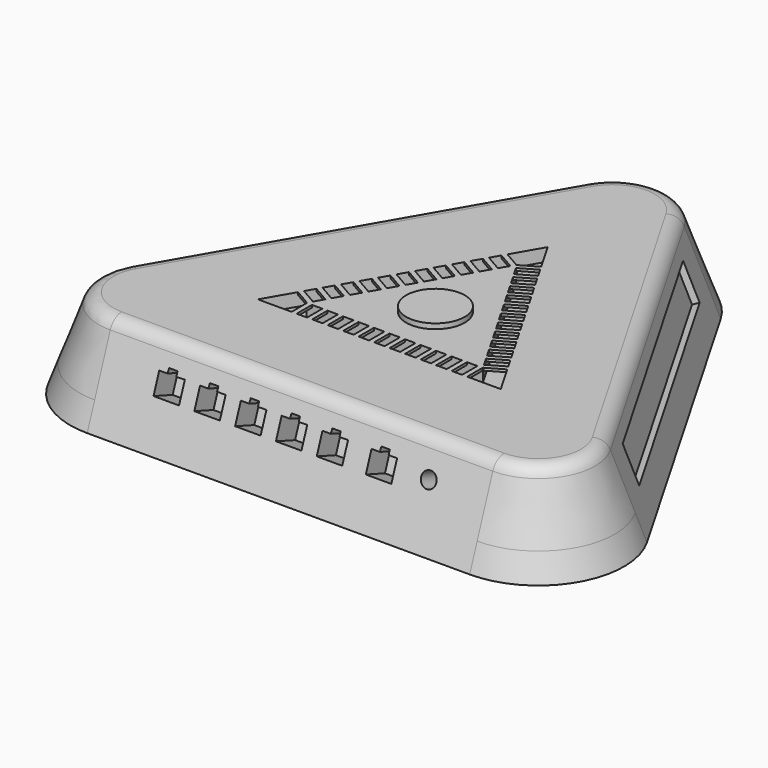
from build123d import *

# Parameters (mm, degrees)
F1_DEPTH      = 25
F1_TAPER      = 20
F1_DEPTH_BACK = 10
F1_TAPER_BACK = -20
F2_R          = 6
F3_R          = 11.5
F4_DEPTH      = 2
F6_R          = 13.9278343954
F7_DEPTH      = 3
F8_R          = 32.5
F9_DEPTH      = 5
F10_R         = 3
F11_DEPTH     = 2
F13_DEPTH     = 5
F15_W         = 1.9796080887
F15_H         = 8.6034480482
F16_DEPTH     = 1
F17_DEPTH     = 10
F19_DEPTH     = 2.5


with BuildPart() as f1:
    # F0 (on Top) → F1 (new body, two sides)
    with BuildSketch(Plane.XY) as f1_sk:
        with BuildLine():
            Line((-75, -73.3012701892), (75, -73.3012701892))
            ThreePointArc((75, -73.3012701892), (100.9807621135, -58.3012701892), (100.9807621135, -28.3012701892))
            Line((100.9807621135, -28.3012701892), (25.9807621135, 101.6025403784))
            ThreePointArc((25.9807621135, 101.6025403784), (0, 116.6025403784), (-25.9807621135, 101.6025403784))
            Line((-25.9807621135, 101.6025403784), (-100.9807621135, -28.3012701892))
            ThreePointArc((-100.9807621135, -28.3012701892), (-100.9807621135, -58.3012701892), (-75, -73.3012701892))
        make_face()
    extrude(amount=F1_DEPTH, taper=F1_TAPER)
    extrude(f1_sk.sketch, amount=-F1_DEPTH_BACK, taper=F1_TAPER_BACK)

    # F2
    f2_edges = [f1.edges().sort_by_distance(p)[0] for p in [
        (-93.100575, -53.751642, 25),
        (0, -64.202014, 25),
        (93.100575, -53.751642, 25),
        (55.600575, 32.101007, 25),
        (0, 107.503285, 25),
        (-55.600575, 32.101007, 25),
    ]]
    fillet(f2_edges, radius=F2_R)

    # F3 (on face) → F4 (join)
    with BuildSketch(Plane.XY.offset(25)):
        Circle(F3_R)
    extrude(amount=F4_DEPTH)

    # F6 (on face) → F7 (join)
    with BuildSketch(Plane(origin=(0, 0, -10), x_dir=(1, 0, 0), z_dir=(0, 0, -1))):
        with Locations((-79.5582754758, 42.91382827)):
            Circle(F6_R)
        with Locations((79.5582754758, 42.91382827)):
            Circle(F6_R)
        with Locations((0, -90.3564020991)):
            Circle(F6_R)
    extrude(amount=F7_DEPTH)

    # F8 (on face) → F9 (cut)
    with BuildSketch(Plane(origin=(0, 0, -10), x_dir=(1, 0, 0), z_dir=(0, 0, -1))):
        Circle(F8_R)
    extrude(amount=-F9_DEPTH, mode=Mode.SUBTRACT)

    # F10 (on face) → F11 (cut)
    with BuildSketch(Plane(origin=(0, -64.7266504456, 23.558574126), x_dir=(1, 0, 0), z_dir=(0, -0.9396926208, 0.3420201433))):
        Polygon((-53.9876961336, -9.3026818497), (-53.9876961336, -17.5021458417), (-43.9876961336, -17.5021458417), (-43.9579116181, -9.2383237345), (-47.2984413058, -9.3026818497), (-47.2984413058, -7.5021458417), (-50.609186478, -7.5021458417), (-50.7396796718, -9.3026818497), align=None)
        Polygon((-34.7396796718, -9.3026818497), (-37.9876961336, -9.3026818497), (-37.9876961336, -17.5021458417), (-27.9876961336, -17.5021458417), (-27.9579116181, -9.2383237345), (-31.2984413058, -9.3026818497), (-31.2984413058, -7.5021458417), (-34.609186478, -7.5021458417), align=None)
        Polygon((-18.7396796718, -9.3026818497), (-21.9876961336, -9.3026818497), (-21.9876961336, -17.5021458417), (-11.9876961336, -17.5021458417), (-11.9579116181, -9.2383237345), (-15.2984413058, -9.3026818497), (-15.2984413058, -7.5021458417), (-18.609186478, -7.5021458417), align=None)
        Polygon((-2.7396796718, -9.3026818497), (-5.9876961336, -9.3026818497), (-5.9876961336, -17.5021458417), (4.0123038664, -17.5021458417), (4.0420883819, -9.2383237345), (0.7015586942, -9.3026818497), (0.7015586942, -7.5021458417), (-2.609186478, -7.5021458417), align=None)
        Polygon((13.2603203282, -9.3026818497), (10.0123038664, -9.3026818497), (10.0123038664, -17.5021458417), (20.0123038664, -17.5021458417), (20.0420883819, -9.2383237345), (16.7015586942, -9.3026818497), (16.7015586942, -7.5021458417), (13.390813522, -7.5021458417), align=None)
        Polygon((32.5083367899, -9.3026819218), (29.2603203282, -9.3026819218), (29.2603203282, -17.5021459138), (39.2603203282, -17.5021459138), (39.2901048437, -9.2383238067), (35.949575156, -9.3026819218), (35.949575156, -7.5021459138), (32.6388299838, -7.5021459138), align=None)
        with Locations((52.4860955775, -12.1968975291)):
            Circle(F10_R)
    extrude(amount=-F11_DEPTH, mode=Mode.SUBTRACT)

    # F3 (on face) → F13 (cut)
    with BuildSketch(Plane.XY.offset(25)):
        Polygon((-47.6313972081, -27.5), (47.6313972081, -27.5), (0, 55), align=None)
        Polygon((0, 40), (34.6410161514, -20), (-34.6410161514, -20), align=None, mode=Mode.SUBTRACT)
    extrude(amount=-F13_DEPTH, mode=Mode.SUBTRACT)

    # F15 (on offset) → F16 (join)
    with BuildSketch(Plane.XY.offset(25)):
        Polygon((-34.415666014, -19.9025444201), (-34.415666014, -19.79204081), (-34.2808202684, -19.79204081), (-33.3725771272, -18.2189175439), (-40.8233816971, -13.9171935197), (-41.8131857415, -15.6315844141), align=None)
        Polygon((-34.2808202684, -19.79204081), (-34.415666014, -19.79204081), (-34.415666014, -19.9025444201), (-34.3623811716, -19.9333084382), align=None)
        Polygon((-32.4360579252, -19.79204081), (-34.2808202684, -19.79204081), (-34.3623811716, -19.9333084382), (-34.415666014, -19.9025444201), (-34.415666014, -28.3954888582), (-32.4360579252, -28.3954888582), align=None)
        with Locations((-27.3458619696, -24.0937648341)):
            Rectangle(F15_W, F15_H)
        with Locations((-21.2658619696, -24.0937648341)):
            Rectangle(F15_W, F15_H)
        with Locations((-15.1858619696, -24.0937648341)):
            Rectangle(F15_W, F15_H)
        with Locations((-9.1058619696, -24.0937648341)):
            Rectangle(F15_W, F15_H)
        with Locations((-3.0258619696, -24.0937648341)):
            Rectangle(F15_W, F15_H)
        with Locations((3.0541380304, -24.0937648341)):
            Rectangle(F15_W, F15_H)
        with Locations((9.1341380304, -24.0937648341)):
            Rectangle(F15_W, F15_H)
        with Locations((15.2141380304, -24.0937648341)):
            Rectangle(F15_W, F15_H)
        with Locations((21.2941380304, -24.0937648341)):
            Rectangle(F15_W, F15_H)
        with Locations((27.3741380304, -24.0937648341)):
            Rectangle(F15_W, F15_H)
        Polygon((34.2808202684, -19.79204081), (34.4439420748, -19.79204081), (34.4439420748, -19.8535688462), (41.7990477111, -15.6070966271), (40.8092436667, -13.8927057328), (33.3584390968, -18.1944297569), align=None)
        Polygon((34.4439420748, -19.8535688462), (34.4439420748, -19.79204081), (34.2808202684, -19.79204081), (34.3482431412, -19.9088206513), align=None)
        Polygon((34.4439420748, -28.3954888582), (34.4439420748, -19.8535688462), (34.3482431412, -19.9088206513), (34.2808202684, -19.79204081), (32.464333986, -19.79204081), (32.464333986, -28.3954888582), align=None)
        Polygon((25.6092436667, 12.4344665423), (18.1584390968, 8.1327425182), (19.1482431412, 6.4183516238), (26.5990477111, 10.7200756479), align=None)
        Polygon((22.5692436667, 17.6999009973), (15.1184390968, 13.3981769732), (16.1082431412, 11.6837860788), (23.5590477111, 15.9855101029), align=None)
        Polygon((10.4092436667, 38.7616388173), (2.9584390968, 34.4599147932), (3.9482431412, 32.7455238988), (11.3990477111, 37.047247923), align=None)
        Polygon((19.5292436667, 22.9653354523), (12.0784390968, 18.6636114282), (13.0682431412, 16.9492205338), (20.5190477111, 21.2509445579), align=None)
        Polygon((0, 39.58408162), (-0.0815609032, 39.7253492482), (-0.0282760608, 39.7561132663), (-7.3833816971, 44.0025854854), (-8.3731857415, 42.288194591), (-0.9223811716, 37.9864705669), align=None)
        Polygon((-0.0282760608, 39.7561132663), (-0.0815609032, 39.7253492482), (0, 39.58408162), (0.0674228728, 39.7008614612), align=None)
        Polygon((7.3692436667, 44.0270732723), (-0.0282760608, 39.7561132663), (0.0674228728, 39.7008614612), (0, 39.58408162), (0.9082431412, 38.0109583539), (8.3590477111, 42.312682378), align=None)
        Polygon((9.0384390968, 23.9290458832), (10.0282431412, 22.2146549888), (17.4790477111, 26.5163790129), (16.4892436667, 28.2307699073), align=None)
        Polygon((31.6892436667, 1.9035976323), (24.2384390968, -2.3981263918), (25.2282431412, -4.1125172862), (32.6790477111, 0.1892067379), align=None)
        Polygon((27.2784390968, -7.6635608469), (28.2682431412, -9.3779517412), (35.7190477111, -5.0762277171), (34.7292436667, -3.3618368227), align=None)
        Polygon((30.3184390968, -12.9289953019), (31.3082431412, -14.6433861962), (38.7590477111, -10.3416621721), (37.7692436667, -8.6272712777), align=None)
        Polygon((21.1984390968, 2.8673080632), (22.1882431412, 1.1529171688), (29.6390477111, 5.4546411929), (28.6492436667, 7.1690320873), align=None)
        Polygon((5.9984390968, 29.1944803382), (6.9882431412, 27.4800894438), (14.4390477111, 31.7818134679), (13.4492436667, 33.4962043623), align=None)
        Polygon((-23.5731857415, 15.9610223159), (-16.1223811716, 11.6592982918), (-15.1325771272, 13.3736891862), (-22.5833816971, 17.6754132103), align=None)
        Polygon((-26.6131857415, 10.6955878609), (-19.1623811716, 6.3938638368), (-18.1725771272, 8.1082547312), (-25.6233816971, 12.4099787553), align=None)
        Polygon((-38.7731857415, -10.3661499591), (-31.3223811716, -14.6678739832), (-30.3325771272, -12.9534830889), (-37.7833816971, -8.6517590647), align=None)
        Polygon((-29.6531857415, 5.4301534059), (-22.2023811716, 1.1284293818), (-21.2125771272, 2.8428202762), (-28.6633816971, 7.1445443003), align=None)
        Polygon((-25.2423811716, -4.1370050732), (-24.2525771272, -2.4226141788), (-31.7033816971, 1.8791098453), (-32.6931857415, 0.1647189509), align=None)
        Polygon((-17.4931857415, 26.491891226), (-10.0423811716, 22.1901672018), (-9.0525771272, 23.9045580962), (-16.5033816971, 28.2062821203), align=None)
        Polygon((-7.0023811716, 27.4556016568), (-6.0125771272, 29.1699925512), (-13.4633816971, 33.4717165753), (-14.4531857415, 31.757325681), align=None)
        Polygon((-3.9623811716, 32.7210361119), (-2.9725771272, 34.4354270062), (-10.4233816971, 38.7371510303), (-11.4131857415, 37.022760136), align=None)
        Polygon((-13.0823811716, 16.9247327468), (-12.0925771272, 18.6391236412), (-19.5433816971, 22.9408476653), (-20.5331857415, 21.2264567709), align=None)
        Polygon((-28.2823811716, -9.4024395282), (-27.2925771272, -7.6880486338), (-34.7433816971, -3.3863246097), (-35.7331857415, -5.1007155041), align=None)
    extrude(amount=-F16_DEPTH)

    # F10 (on face) → F17 (cut)
    with BuildSketch(Plane(origin=(0, -64.7266504456, 23.558574126), x_dir=(1, 0, 0), z_dir=(0, -0.9396926208, 0.3420201433))):
        Polygon((-53.9876961336, -9.3026818497), (-53.9876961336, -17.5021458417), (-43.9876961336, -17.5021458417), (-43.9579116181, -9.2383237345), (-47.2984413058, -9.3026818497), (-47.2984413058, -7.5021458417), (-50.609186478, -7.5021458417), (-50.7396796718, -9.3026818497), align=None)
        Polygon((-34.7396796718, -9.3026818497), (-37.9876961336, -9.3026818497), (-37.9876961336, -17.5021458417), (-27.9876961336, -17.5021458417), (-27.9579116181, -9.2383237345), (-31.2984413058, -9.3026818497), (-31.2984413058, -7.5021458417), (-34.609186478, -7.5021458417), align=None)
        Polygon((-18.7396796718, -9.3026818497), (-21.9876961336, -9.3026818497), (-21.9876961336, -17.5021458417), (-11.9876961336, -17.5021458417), (-11.9579116181, -9.2383237345), (-15.2984413058, -9.3026818497), (-15.2984413058, -7.5021458417), (-18.609186478, -7.5021458417), align=None)
        Polygon((-2.7396796718, -9.3026818497), (-5.9876961336, -9.3026818497), (-5.9876961336, -17.5021458417), (4.0123038664, -17.5021458417), (4.0420883819, -9.2383237345), (0.7015586942, -9.3026818497), (0.7015586942, -7.5021458417), (-2.609186478, -7.5021458417), align=None)
        Polygon((13.2603203282, -9.3026818497), (10.0123038664, -9.3026818497), (10.0123038664, -17.5021458417), (20.0123038664, -17.5021458417), (20.0420883819, -9.2383237345), (16.7015586942, -9.3026818497), (16.7015586942, -7.5021458417), (13.390813522, -7.5021458417), align=None)
        Polygon((32.5083367899, -9.3026819218), (29.2603203282, -9.3026819218), (29.2603203282, -17.5021459138), (39.2603203282, -17.5021459138), (39.2901048437, -9.2383238067), (35.949575156, -9.3026819218), (35.949575156, -7.5021459138), (32.6388299838, -7.5021459138), align=None)
        with Locations((52.4860955775, -12.1968975291)):
            Circle(F10_R)
    extrude(amount=-F17_DEPTH, mode=Mode.SUBTRACT)

    # F18 (on face) → F19 (cut)
    with BuildSketch(Plane(origin=(56.0549235878, 32.3633252228, 23.558574126), x_dir=(-0.4331471005, 0.882748234, -0.1820416017), z_dir=(0.8137976813, 0.4698463104, 0.3420201433))):
        Polygon((61.7270778404, 4.3735968834), (-58.7563835947, -19.4177206509), (-55.8505142017, -34.133559841), (64.6329472334, -10.3422423067), align=None)
    extrude(amount=-F19_DEPTH, mode=Mode.SUBTRACT)


solid = f1.part
